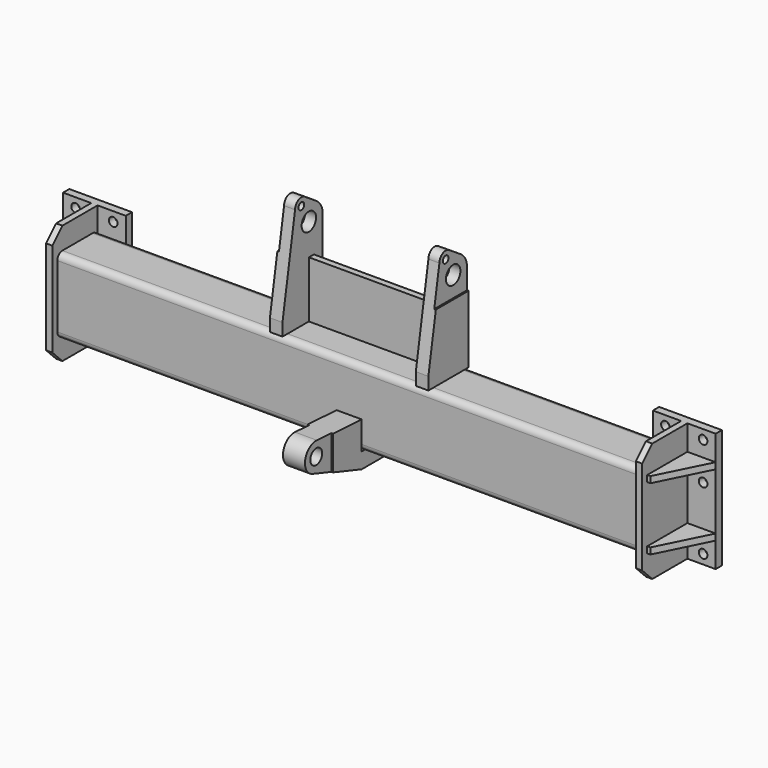
from build123d import *

# Parameters (mm, degrees)
F1_DEPTH  = 1181.1
F2_W      = 228.6
F2_H      = 482.6
F3_DEPTH  = 25.4
F4_SIZE   = 50.8
F5_W      = 254
F5_H      = 482.6
F5_R      = 17.526
F6_DEPTH  = 31.75
F7_W      = 114.3
F7_H      = 25.4
F8_DEPTH  = 203.2
F10_DEPTH = 381.001
F13_W     = 25.4
F13_H     = 228.6
F14_DEPTH = 269.875
F15_R     = 14.2875
F15_R_2   = 36.5125
F15_W     = 25.4
F15_H     = 228.6
F16_DEPTH = 50.8
F17_W     = 361.3794893026
F17_H     = 323.3922393799
F18_DEPTH = 6.35
F20_R     = 30.1625
F21_DEPTH = 50.8
F23_DEPTH = 6.35


with BuildPart() as f1:
    # F0 (on Right) → F1 (new body, symmetric)
    with BuildSketch(Plane.YZ):
        with BuildLine():
            Line((76.2, 152.4), (-76.2, 152.4))
            ThreePointArc((-76.2, 152.4), (-94.1605122421, 144.9605122421), (-101.6, 127))
            Line((-101.6, 127), (-101.6, -127))
            ThreePointArc((-101.6, -127), (-94.1605122421, -144.9605122421), (-76.2, -152.4))
            Line((-76.2, -152.4), (76.2, -152.4))
            ThreePointArc((76.2, -152.4), (94.1605122421, -144.9605122421), (101.6, -127))
            Line((101.6, -127), (101.6, 127))
            ThreePointArc((101.6, 127), (94.1605122421, 144.9605122421), (76.2, 152.4))
        make_face()
        with BuildLine():
            ThreePointArc((-88.9, 127), (-85.1802561211, 135.9802561211), (-76.2, 139.7))
            Line((-76.2, 139.7), (76.2, 139.7))
            ThreePointArc((76.2, 139.7), (85.1802561211, 135.9802561211), (88.9, 127))
            Line((88.9, 127), (88.9, -127))
            ThreePointArc((88.9, -127), (85.1802561211, -135.9802561211), (76.2, -139.7))
            Line((76.2, -139.7), (-76.2, -139.7))
            ThreePointArc((-76.2, -139.7), (-85.1802561211, -135.9802561211), (-88.9, -127))
            Line((-88.9, -127), (-88.9, 127))
        make_face(mode=Mode.SUBTRACT)
    extrude(amount=F1_DEPTH, both=True)

    # F2 (on face) → F3 (join)
    with BuildSketch(Plane.YZ.offset(1181.1)):
        with Locations((-12.7, 0)):
            Rectangle(F2_W, F2_H)
    extrude(amount=F3_DEPTH)

    # F4
    f4_edges = [f1.edges().sort_by_distance(p)[0] for p in [
        (1193.8, -127, 241.3),
        (1193.8, -127, -241.3),
    ]]
    chamfer(f4_edges, length=F4_SIZE)

    # F5 (on face) → F6 (join)
    with BuildSketch(Plane(origin=(0, 101.6, 0), x_dir=(-1, 0, 0), z_dir=(0, 1, 0))):
        with Locations((-1193.8, 0)):
            Rectangle(F5_W, F5_H)
        with Locations((-1270, -203.2)):
            Circle(F5_R, mode=Mode.SUBTRACT)
        with Locations((-1117.6, -203.2)):
            Circle(F5_R, mode=Mode.SUBTRACT)
        with Locations((-1270, 50.8)):
            Circle(F5_R, mode=Mode.SUBTRACT)
        with Locations((-1270, 203.2)):
            Circle(F5_R, mode=Mode.SUBTRACT)
        with Locations((-1117.6, 203.2)):
            Circle(F5_R, mode=Mode.SUBTRACT)
    extrude(amount=F6_DEPTH)

    # F7 (on face) → F8 (join)
    with BuildSketch(Plane.XZ.offset(-101.6)):
        with Locations((1263.65, 127)):
            Rectangle(F7_W, F7_H)
        with Locations((1263.65, -127)):
            Rectangle(F7_W, F7_H)
    extrude(amount=F8_DEPTH)

    # F9 (on face) → F10 (cut, through all)
    with BuildSketch(Plane.XY.offset(139.7)):
        Polygon((1219.2, -101.6), (1320.8, -101.6), (1320.8, 101.6), align=None)
    extrude(amount=-F10_DEPTH, mode=Mode.SUBTRACT)


with BuildPart() as f11_1:
    # F11: instance of F1
    add(f1.part.mirror(Plane.YZ))


with BuildPart() as f1_1:
    add(f1.part)

    # F12: union F11_1
    add(f11_1.part)

    # F13 (on Right) → F14 (join, symmetric)
    with BuildSketch(Plane.YZ):
        with Locations((44.45, 266.7)):
            Rectangle(F13_W, F13_H)
    extrude(amount=F14_DEPTH, both=True)

    # F15 (on face) → F16 (join)
    with BuildSketch(Plane.YZ.offset(269.875)):
        with BuildLine():
            Line((57.15, 152.4), (101.6, 152.4))
            Line((101.6, 152.4), (101.6, 508))
            ThreePointArc((101.6, 508), (93.2355821831, 541.1443160075), (70.1455781359, 566.3506819121))
            Line((70.1455781359, 566.3506819121), (11.1025355163, 605.2018432352))
            ThreePointArc((11.1025355163, 605.2018432352), (-21.4155981852, 606.6267979039), (-38.1, 578.6788060024))
            Line((-38.1, 578.6788060024), (-101.6, 203.2))
            Line((-101.6, 203.2), (-101.6, 152.4))
            Line((-101.6, 152.4), (31.75, 152.4))
            Line((31.75, 152.4), (31.75, 381))
            Line((31.75, 381), (57.15, 381))
            Line((57.15, 381), (57.15, 152.4))
        make_face()
        with Locations((-6.35, 578.6788060024)):
            Circle(F15_R, mode=Mode.SUBTRACT)
        with Locations((31.75, 508)):
            Circle(F15_R_2, mode=Mode.SUBTRACT)
        with Locations((44.45, 266.7)):
            Rectangle(F15_W, F15_H)
    extrude(amount=F16_DEPTH)

    # F17 (on face) → F18 (cut)
    with BuildSketch(Plane.YZ.offset(320.675)):
        with Locations((24.2072567344, 587.1461196899)):
            Rectangle(F17_W, F17_H)
    extrude(amount=-F18_DEPTH, mode=Mode.SUBTRACT)


with BuildPart() as f19_1:
    # F19: instance of F1
    add(f1_1.part.mirror(Plane.YZ))


with BuildPart() as f1_2:
    add(f1_1.part)

    add(f19_1.part)  # F21 merges F19_1
    # F20 (on Right) → F21 (join, symmetric)
    with BuildSketch(Plane.YZ):
        with BuildLine():
            Line((-101.6, -215.9), (76.2, -215.9))
            Line((76.2, -215.9), (76.2, -152.4))
            Line((76.2, -152.4), (-101.6, -152.4))
            Line((-101.6, -152.4), (-101.6, -139.7))
            Line((-101.6, -139.7), (-101.6, -127))
            Line((-101.6, -127), (-101.6, -38.1))
            Line((-101.6, -38.1), (-320.5653923257, -25.4944669429))
            ThreePointArc((-320.5653923257, -25.4944669429), (-379.9951543899, -71.8802231262), (-341.724064813, -136.8329651646))
            Line((-341.724064813, -136.8329651646), (-101.6, -215.9))
        make_face()
        with Locations((-323.85, -82.55)):
            Circle(F20_R, mode=Mode.SUBTRACT)
    extrude(amount=F21_DEPTH, both=True)


with BuildPart() as f23:
    # F22 (on face) → F23 (new body)
    with BuildSketch(Plane.YZ.offset(50.8)):
        Polygon((-247.65, -212.9706889391), (-247.65, -82.55), (-247.65, 21.7781551182), (-439.1066730022, 21.7781551182), (-439.1066730022, -212.9706889391), align=None)
    extrude(amount=-F23_DEPTH)


with BuildPart() as f24_1:
    # F24: instance of F23
    add(f23.part.mirror(Plane.YZ))


with BuildPart() as f1_3:
    add(f1_2.part)

    # F25: cut F24_1, F23
    add(f24_1.part, mode=Mode.SUBTRACT)
    add(f23.part, mode=Mode.SUBTRACT)


solid = f1_3.part
